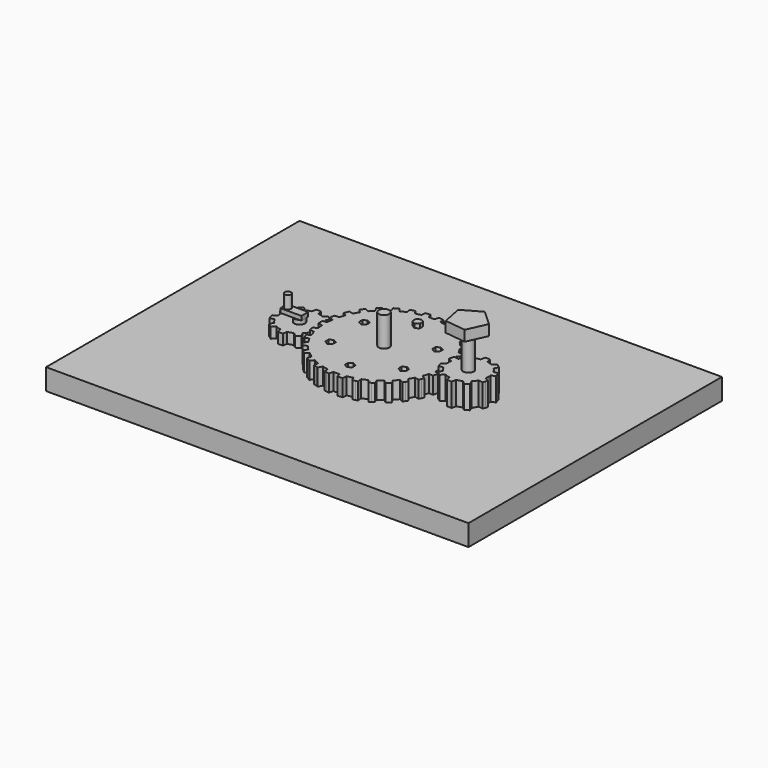
from build123d import *

# Parameters (mm, degrees)
F0_W      = 200
F0_H      = 150
F1_DEPTH  = 10
F2_R      = 4
F2_R_2    = 2.5
F3_DEPTH  = 3
F4_DEPTH  = 10
F6_DEPTH  = 5
F7_DEPTH  = 25
F8_DEPTH  = 30
F10_DEPTH = 11
F11_W     = 10
F11_H     = 4
F12_DEPTH = 2
F13_R     = 1.5
F14_DEPTH = 6
F16_DEPTH = 5
F18_DEPTH = 8
F20_DEPTH = 3
F21_DEPTH = 5


with BuildPart() as f1:
    # F0 (on Top) → F1 (new body)
    with BuildSketch(Plane.XY):
        Rectangle(F0_W, F0_H)
    extrude(amount=F1_DEPTH)

    # F2 (on face) → F3 (join)
    with BuildSketch(Plane.XY.offset(10)):
        Circle(F2_R)
        Circle(F2_R_2, mode=Mode.SUBTRACT)
        with Locations((-40, 0)):
            Circle(F2_R)
        with Locations((-40, 0)):
            Circle(F2_R_2, mode=Mode.SUBTRACT)
        with Locations((40, 0)):
            Circle(F2_R)
        with Locations((40, 0)):
            Circle(F2_R_2, mode=Mode.SUBTRACT)
    extrude(amount=F3_DEPTH)


with BuildPart() as f4:
    # F4 (new): a face of the model
    f4_faces = [f1.part.faces().sort_by_distance(p)[0] for p in [
        (-40, 0, 10),
    ]]
    extrude(f4_faces, amount=F4_DEPTH)

    # F5 (on face) → F6 (join)
    with BuildSketch(Plane.XY.offset(13)):
        with BuildLine():
            ThreePointArc((-30.7270362333, -1.3794085621), (-30.6505438577, -0.6915886375), (-30.625, 0))
            ThreePointArc((-30.625, 0), (-30.6505438577, 0.6915886375), (-30.7270362333, 1.3794085621))
            ThreePointArc((-30.7270362333, 1.3794085621), (-31.0838451597, 2.8970343223), (-31.6872187148, 4.3345463782))
            ThreePointArc((-31.6872187148, 4.3345463782), (-32.4154656777, 5.5104867402), (-33.3088107342, 6.566476316))
            ThreePointArc((-33.3088107342, 6.566476316), (-34.4895132598, 7.5845343223), (-35.8226011062, 8.3928519278))
            ThreePointArc((-35.8226011062, 8.3928519278), (-37.1029656777, 8.9161548403), (-38.4463921095, 9.2453733036))
            ThreePointArc((-38.4463921095, 9.2453733036), (-40, 9.375), (-41.5536078905, 9.2453733036))
            ThreePointArc((-41.5536078905, 9.2453733036), (-42.8970343223, 8.9161548403), (-44.1773988938, 8.3928519278))
            ThreePointArc((-44.1773988938, 8.3928519278), (-45.5104867402, 7.5845343223), (-46.6911892658, 6.566476316))
            ThreePointArc((-46.6911892658, 6.566476316), (-47.5845343223, 5.5104867402), (-48.3127812852, 4.3345463782))
            ThreePointArc((-48.3127812852, 4.3345463782), (-48.9161548403, 2.8970343223), (-49.2729637667, 1.3794085621))
            ThreePointArc((-49.2729637667, 1.3794085621), (-49.375, 0), (-49.2729637667, -1.3794085621))
            ThreePointArc((-49.2729637667, -1.3794085621), (-48.9161548403, -2.8970343223), (-48.3127812852, -4.3345463782))
            ThreePointArc((-48.3127812852, -4.3345463782), (-47.5845343223, -5.5104867402), (-46.6911892658, -6.566476316))
            ThreePointArc((-46.6911892658, -6.566476316), (-45.5104867402, -7.5845343223), (-44.1773988938, -8.3928519278))
            ThreePointArc((-44.1773988938, -8.3928519278), (-42.8970343223, -8.9161548403), (-41.5536078905, -9.2453733036))
            ThreePointArc((-41.5536078905, -9.2453733036), (-40, -9.375), (-38.4463921095, -9.2453733036))
            ThreePointArc((-38.4463921095, -9.2453733036), (-37.1029656777, -8.9161548403), (-35.8226011062, -8.3928519278))
            ThreePointArc((-35.8226011062, -8.3928519278), (-34.4895132598, -7.5845343223), (-33.3088107342, -6.566476316))
            ThreePointArc((-33.3088107342, -6.566476316), (-32.4154656777, -5.5104867402), (-31.6872187148, -4.3345463782))
            ThreePointArc((-31.6872187148, -4.3345463782), (-31.0838451597, -2.8970343223), (-30.7270362333, -1.3794085621))
        make_face()
        with BuildLine():
            ThreePointArc((-31.6872187148, 4.3345463782), (-31.0838451597, 2.8970343223), (-30.7270362333, 1.3794085621))
            Line((-30.7270362333, 1.3794085621), (-28.8176800574, 2.3946312492))
            Line((-28.8176800574, 2.3946312492), (-29.1817321271, 3.515068311))
            Line((-29.1817321271, 3.515068311), (-29.5457841969, 4.6355053728))
            Line((-29.5457841969, 4.6355053728), (-31.6872187148, 4.3345463782))
        make_face()
        with BuildLine():
            Line((-28.8176800574, -2.3946312492), (-30.7270362333, -1.3794085621))
            ThreePointArc((-30.7270362333, -1.3794085621), (-31.0838451597, -2.8970343223), (-31.6872187148, -4.3345463782))
            Line((-31.6872187148, -4.3345463782), (-29.5457841969, -4.6355053728))
            Line((-29.5457841969, -4.6355053728), (-29.1817321271, -3.515068311))
            Line((-29.1817321271, -3.515068311), (-28.8176800574, -2.3946312492))
        make_face()
        with BuildLine():
            ThreePointArc((-35.8226011062, 8.3928519278), (-34.4895132598, 7.5845343223), (-33.3088107342, 6.566476316))
            Line((-33.3088107342, 6.566476316), (-32.3608420629, 8.5101001246))
            Line((-32.3608420629, 8.5101001246), (-33.3139427552, 9.202568311))
            Line((-33.3139427552, 9.202568311), (-34.2670434475, 9.8950364974))
            Line((-34.2670434475, 9.8950364974), (-35.8226011062, 8.3928519278))
        make_face()
        with BuildLine():
            Line((-32.3608420629, -8.5101001246), (-33.3088107342, -6.566476316))
            ThreePointArc((-33.3088107342, -6.566476316), (-34.4895132598, -7.5845343223), (-35.8226011062, -8.3928519278))
            Line((-35.8226011062, -8.3928519278), (-34.2670434475, -9.8950364974))
            Line((-34.2670434475, -9.8950364974), (-33.3139427552, -9.202568311))
            Line((-33.3139427552, -9.202568311), (-32.3608420629, -8.5101001246))
        make_face()
        with BuildLine():
            ThreePointArc((-41.5536078905, 9.2453733036), (-40, 9.375), (-38.4463921095, 9.2453733036))
            Line((-38.4463921095, 9.2453733036), (-38.8219027549, 11.375))
            Line((-38.8219027549, 11.375), (-40, 11.375))
            Line((-40, 11.375), (-41.1780972451, 11.375))
            Line((-41.1780972451, 11.375), (-41.5536078905, 9.2453733036))
        make_face()
        with BuildLine():
            Line((-38.8219027549, -11.375), (-38.4463921095, -9.2453733036))
            ThreePointArc((-38.4463921095, -9.2453733036), (-40, -9.375), (-41.5536078905, -9.2453733036))
            Line((-41.5536078905, -9.2453733036), (-41.1780972451, -11.375))
            Line((-41.1780972451, -11.375), (-40, -11.375))
            Line((-40, -11.375), (-38.8219027549, -11.375))
        make_face()
        with BuildLine():
            ThreePointArc((-46.6911892658, 6.566476316), (-45.5104867402, 7.5845343223), (-44.1773988938, 8.3928519278))
            Line((-44.1773988938, 8.3928519278), (-45.7329565525, 9.8950364974))
            Line((-45.7329565525, 9.8950364974), (-46.6860572448, 9.202568311))
            Line((-46.6860572448, 9.202568311), (-47.6391579371, 8.5101001246))
            Line((-47.6391579371, 8.5101001246), (-46.6911892658, 6.566476316))
        make_face()
        with BuildLine():
            Line((-45.7329565525, -9.8950364974), (-44.1773988938, -8.3928519278))
            ThreePointArc((-44.1773988938, -8.3928519278), (-45.5104867402, -7.5845343223), (-46.6911892658, -6.566476316))
            Line((-46.6911892658, -6.566476316), (-47.6391579371, -8.5101001246))
            Line((-47.6391579371, -8.5101001246), (-46.6860572448, -9.202568311))
            Line((-46.6860572448, -9.202568311), (-45.7329565525, -9.8950364974))
        make_face()
        with BuildLine():
            ThreePointArc((-49.2729637667, 1.3794085621), (-48.9161548403, 2.8970343223), (-48.3127812852, 4.3345463782))
            Line((-48.3127812852, 4.3345463782), (-50.4542158031, 4.6355053728))
            Line((-50.4542158031, 4.6355053728), (-50.8182678729, 3.515068311))
            Line((-50.8182678729, 3.515068311), (-51.1823199426, 2.3946312492))
            Line((-51.1823199426, 2.3946312492), (-49.2729637667, 1.3794085621))
        make_face()
        with BuildLine():
            Line((-50.4542158031, -4.6355053728), (-48.3127812852, -4.3345463782))
            ThreePointArc((-48.3127812852, -4.3345463782), (-48.9161548403, -2.8970343223), (-49.2729637667, -1.3794085621))
            Line((-49.2729637667, -1.3794085621), (-51.1823199426, -2.3946312492))
            Line((-51.1823199426, -2.3946312492), (-50.8182678729, -3.515068311))
            Line((-50.8182678729, -3.515068311), (-50.4542158031, -4.6355053728))
        make_face()
    extrude(amount=F6_DEPTH)

    # F11 (on face) → F12 (join)
    with BuildSketch(Plane.XY.offset(20)):
        with Locations((-42.5, 0)):
            Rectangle(F11_W, F11_H)
    extrude(amount=F12_DEPTH)

    # F13 (on face) → F14 (join)
    with BuildSketch(Plane.XY.offset(22)):
        with Locations((-45.5, 0)):
            Circle(F13_R)
    extrude(amount=F14_DEPTH)


with BuildPart() as f7:
    # F7 (new): a face of the model
    f7_faces = [f1.part.faces().sort_by_distance(p)[0] for p in [
        (0, 0, 10),
    ]]
    extrude(f7_faces, amount=F7_DEPTH)

    # F17 (on face) → F18 (join)
    with BuildSketch(Plane.XY.offset(13)):
        with BuildLine():
            ThreePointArc((28.0829066802, -1.5381733945), (28.1144747006, -0.7693746225), (28.125, 0))
            ThreePointArc((28.125, 0), (28.1144747006, 0.7693746225), (28.0829066802, 1.5381733945))
            ThreePointArc((28.0829066802, 1.5381733945), (27.9709283072, 2.9398630294), (27.7890320221, 4.3342039956))
            ThreePointArc((27.7890320221, 4.3342039956), (27.5104012706, 5.8475163042), (27.1494235596, 7.3433252263))
            ThreePointArc((27.1494235596, 7.3433252263), (26.7484645208, 8.6911029668), (26.280643318, 10.0171558733))
            ThreePointArc((26.280643318, 10.0171558733), (25.6934659962, 11.4394680865), (25.0293803521, 12.8275385085))
            ThreePointArc((25.0293803521, 12.8275385085), (24.3569644814, 14.0625), (23.6236643925, 15.2623099717))
            ThreePointArc((23.6236643925, 15.2623099717), (22.7536029668, 16.5314602207), (21.815433119, 17.7511268046))
            ThreePointArc((21.815433119, 17.7511268046), (20.9009482166, 18.8192983038), (19.934217974, 19.8404278876))
            ThreePointArc((19.934217974, 19.8404278876), (18.8192983038, 20.9009482166), (17.6480467764, 21.8989056799))
            ThreePointArc((17.6480467764, 21.8989056799), (16.5314602207, 22.7536029668), (15.3735505752, 23.5514238999))
            ThreePointArc((15.3735505752, 23.5514238999), (14.0625, 24.3569644814), (12.709356105, 25.0895972944))
            ThreePointArc((12.709356105, 25.0895972944), (11.4394680865, 25.6934659962), (10.1409852457, 26.2331096755))
            ThreePointArc((10.1409852457, 26.2331096755), (8.6911029668, 26.7484645208), (7.2152055856, 27.1837531139))
            ThreePointArc((7.2152055856, 27.1837531139), (5.8475163042, 27.5104012706), (4.4652101991, 27.7682826779))
            ThreePointArc((4.4652101991, 27.7682826779), (2.9398630294, 27.9709283072), (1.4057159597, 28.0898484802))
            ThreePointArc((1.4057159597, 28.0898484802), (0, 28.125), (-1.4057159597, 28.0898484802))
            ThreePointArc((-1.4057159597, 28.0898484802), (-2.9398630294, 27.9709283072), (-4.4652101991, 27.7682826779))
            ThreePointArc((-4.4652101991, 27.7682826779), (-5.8475163042, 27.5104012706), (-7.2152055856, 27.1837531139))
            ThreePointArc((-7.2152055856, 27.1837531139), (-8.6911029668, 26.7484645208), (-10.1409852457, 26.2331096755))
            ThreePointArc((-10.1409852457, 26.2331096755), (-11.4394680865, 25.6934659962), (-12.709356105, 25.0895972944))
            ThreePointArc((-12.709356105, 25.0895972944), (-14.0625, 24.3569644814), (-15.3735505752, 23.5514238999))
            ThreePointArc((-15.3735505752, 23.5514238999), (-16.5314602207, 22.7536029668), (-17.6480467764, 21.8989056799))
            ThreePointArc((-17.6480467764, 21.8989056799), (-18.8192983038, 20.9009482166), (-19.934217974, 19.8404278876))
            ThreePointArc((-19.934217974, 19.8404278876), (-20.9009482166, 18.8192983038), (-21.815433119, 17.7511268046))
            ThreePointArc((-21.815433119, 17.7511268046), (-22.7536029668, 16.5314602207), (-23.6236643925, 15.2623099717))
            ThreePointArc((-23.6236643925, 15.2623099717), (-24.3569644814, 14.0625), (-25.0293803521, 12.8275385085))
            ThreePointArc((-25.0293803521, 12.8275385085), (-25.6934659962, 11.4394680865), (-26.280643318, 10.0171558733))
            ThreePointArc((-26.280643318, 10.0171558733), (-26.7484645208, 8.6911029668), (-27.1494235596, 7.3433252263))
            ThreePointArc((-27.1494235596, 7.3433252263), (-27.5104012706, 5.8475163042), (-27.7890320221, 4.3342039956))
            ThreePointArc((-27.7890320221, 4.3342039956), (-27.9709283072, 2.9398630294), (-28.0829066802, 1.5381733945))
            ThreePointArc((-28.0829066802, 1.5381733945), (-28.125, 0), (-28.0829066802, -1.5381733945))
            ThreePointArc((-28.0829066802, -1.5381733945), (-27.9709283072, -2.9398630294), (-27.7890320221, -4.3342039956))
            ThreePointArc((-27.7890320221, -4.3342039956), (-27.5104012706, -5.8475163042), (-27.1494235596, -7.3433252263))
            ThreePointArc((-27.1494235596, -7.3433252263), (-26.7484645208, -8.6911029668), (-26.280643318, -10.0171558733))
            ThreePointArc((-26.280643318, -10.0171558733), (-25.6934659962, -11.4394680865), (-25.0293803521, -12.8275385085))
            ThreePointArc((-25.0293803521, -12.8275385085), (-24.3569644814, -14.0625), (-23.6236643925, -15.2623099717))
            ThreePointArc((-23.6236643925, -15.2623099717), (-22.7536029668, -16.5314602207), (-21.815433119, -17.7511268046))
            ThreePointArc((-21.815433119, -17.7511268046), (-20.9009482166, -18.8192983038), (-19.934217974, -19.8404278876))
            ThreePointArc((-19.934217974, -19.8404278876), (-18.8192983038, -20.9009482166), (-17.6480467764, -21.8989056799))
            ThreePointArc((-17.6480467764, -21.8989056799), (-16.5314602207, -22.7536029668), (-15.3735505752, -23.5514238999))
            ThreePointArc((-15.3735505752, -23.5514238999), (-14.0625, -24.3569644814), (-12.709356105, -25.0895972944))
            ThreePointArc((-12.709356105, -25.0895972944), (-11.4394680865, -25.6934659962), (-10.1409852457, -26.2331096755))
            ThreePointArc((-10.1409852457, -26.2331096755), (-8.6911029668, -26.7484645208), (-7.2152055856, -27.1837531139))
            ThreePointArc((-7.2152055856, -27.1837531139), (-5.8475163042, -27.5104012706), (-4.4652101991, -27.7682826779))
            ThreePointArc((-4.4652101991, -27.7682826779), (-2.9398630294, -27.9709283072), (-1.4057159597, -28.0898484802))
            ThreePointArc((-1.4057159597, -28.0898484802), (0, -28.125), (1.4057159597, -28.0898484802))
            ThreePointArc((1.4057159597, -28.0898484802), (2.9398630294, -27.9709283072), (4.4652101991, -27.7682826779))
            ThreePointArc((4.4652101991, -27.7682826779), (5.8475163042, -27.5104012706), (7.2152055856, -27.1837531139))
            ThreePointArc((7.2152055856, -27.1837531139), (8.6911029668, -26.7484645208), (10.1409852457, -26.2331096755))
            ThreePointArc((10.1409852457, -26.2331096755), (11.4394680865, -25.6934659962), (12.709356105, -25.0895972944))
            ThreePointArc((12.709356105, -25.0895972944), (14.0625, -24.3569644814), (15.3735505752, -23.5514238999))
            ThreePointArc((15.3735505752, -23.5514238999), (16.5314602207, -22.7536029668), (17.6480467764, -21.8989056799))
            ThreePointArc((17.6480467764, -21.8989056799), (18.8192983038, -20.9009482166), (19.934217974, -19.8404278876))
            ThreePointArc((19.934217974, -19.8404278876), (20.9009482166, -18.8192983038), (21.815433119, -17.7511268046))
            ThreePointArc((21.815433119, -17.7511268046), (22.7536029668, -16.5314602207), (23.6236643925, -15.2623099717))
            ThreePointArc((23.6236643925, -15.2623099717), (24.3569644814, -14.0625), (25.0293803521, -12.8275385085))
            ThreePointArc((25.0293803521, -12.8275385085), (25.6934659962, -11.4394680865), (26.280643318, -10.0171558733))
            ThreePointArc((26.280643318, -10.0171558733), (26.7484645208, -8.6911029668), (27.1494235596, -7.3433252263))
            ThreePointArc((27.1494235596, -7.3433252263), (27.5104012706, -5.8475163042), (27.7890320221, -4.3342039956))
            ThreePointArc((27.7890320221, -4.3342039956), (27.9709283072, -2.9398630294), (28.0829066802, -1.5381733945))
        make_face()
        with BuildLine():
            ThreePointArc((28.0829066802, 1.5381733945), (28.1144747006, 0.7693746225), (28.125, 0))
            ThreePointArc((28.125, 0), (28.1144747006, -0.7693746225), (28.0829066802, -1.5381733945))
            Line((28.0829066802, -1.5381733945), (30.125, -1.1780972451))
            Line((30.125, -1.1780972451), (30.125, 0))
            Line((30.125, 0), (30.125, 1.1780972451))
            Line((30.125, 1.1780972451), (28.0829066802, 1.5381733945))
        make_face()
        with BuildLine():
            ThreePointArc((27.1494235596, 7.3433252263), (27.5104012706, 5.8475163042), (27.7890320221, 4.3342039956))
            Line((27.7890320221, 4.3342039956), (29.7116366623, 5.1109866922))
            Line((29.7116366623, 5.1109866922), (29.4666964721, 6.2633396859))
            Line((29.4666964721, 6.2633396859), (29.2217562819, 7.4156926796))
            Line((29.2217562819, 7.4156926796), (27.1494235596, 7.3433252263))
        make_face()
        with BuildLine():
            Line((29.7116366623, -5.1109866922), (27.7890320221, -4.3342039956))
            ThreePointArc((27.7890320221, -4.3342039956), (27.5104012706, -5.8475163042), (27.1494235596, -7.3433252263))
            Line((27.1494235596, -7.3433252263), (29.2217562819, -7.4156926796))
            Line((29.2217562819, -7.4156926796), (29.4666964721, -6.2633396859))
            Line((29.4666964721, -6.2633396859), (29.7116366623, -5.1109866922))
        make_face()
        with BuildLine():
            ThreePointArc((25.0293803521, 12.8275385085), (25.6934659962, 11.4394680865), (26.280643318, 10.0171558733))
            Line((26.280643318, 10.0171558733), (27.9997322302, 11.1766959857))
            Line((27.9997322302, 11.1766959857), (27.5205569115, 12.2529413727))
            Line((27.5205569115, 12.2529413727), (27.0413815928, 13.3291867596))
            Line((27.0413815928, 13.3291867596), (25.0293803521, 12.8275385085))
        make_face()
        with BuildLine():
            Line((27.9997322302, -11.1766959857), (26.280643318, -10.0171558733))
            ThreePointArc((26.280643318, -10.0171558733), (25.6934659962, -11.4394680865), (25.0293803521, -12.8275385085))
            Line((25.0293803521, -12.8275385085), (27.0413815928, -13.3291867596))
            Line((27.0413815928, -13.3291867596), (27.5205569115, -12.2529413727))
            Line((27.5205569115, -12.2529413727), (27.9997322302, -11.1766959857))
        make_face()
        with BuildLine():
            ThreePointArc((21.815433119, 17.7511268046), (22.7536029668, 16.5314602207), (23.6236643925, 15.2623099717))
            Line((23.6236643925, 15.2623099717), (25.064105142, 16.753930033))
            Line((25.064105142, 16.753930033), (24.3716369555, 17.7070307253))
            Line((24.3716369555, 17.7070307253), (23.6791687691, 18.6601314176))
            Line((23.6791687691, 18.6601314176), (21.815433119, 17.7511268046))
        make_face()
        with BuildLine():
            Line((25.064105142, -16.753930033), (23.6236643925, -15.2623099717))
            ThreePointArc((23.6236643925, -15.2623099717), (22.7536029668, -16.5314602207), (21.815433119, -17.7511268046))
            Line((21.815433119, -17.7511268046), (23.6791687691, -18.6601314176))
            Line((23.6791687691, -18.6601314176), (24.3716369555, -17.7070307253))
            Line((24.3716369555, -17.7070307253), (25.064105142, -16.753930033))
        make_face()
        with BuildLine():
            ThreePointArc((17.6480467764, 21.8989056799), (18.8192983038, 20.9009482166), (19.934217974, 19.8404278876))
            Line((19.934217974, 19.8404278876), (21.0330563882, 21.5989369435))
            Line((21.0330563882, 21.5989369435), (20.1575595166, 22.3872378675))
            Line((20.1575595166, 22.3872378675), (19.282062645, 23.1755387915))
            Line((19.282062645, 23.1755387915), (17.6480467764, 21.8989056799))
        make_face()
        with BuildLine():
            Line((21.0330563882, -21.5989369435), (19.934217974, -19.8404278876))
            ThreePointArc((19.934217974, -19.8404278876), (18.8192983038, -20.9009482166), (17.6480467764, -21.8989056799))
            Line((17.6480467764, -21.8989056799), (19.282062645, -23.1755387915))
            Line((19.282062645, -23.1755387915), (20.1575595166, -22.3872378675))
            Line((20.1575595166, -22.3872378675), (21.0330563882, -21.5989369435))
        make_face()
        with BuildLine():
            ThreePointArc((12.709356105, 25.0895972944), (14.0625, 24.3569644814), (15.3735505752, 23.5514238999))
            Line((15.3735505752, 23.5514238999), (16.0827621424, 25.4999666665))
            Line((16.0827621424, 25.4999666665), (15.0625, 26.089015289))
            Line((15.0625, 26.089015289), (14.0422378576, 26.6780639116))
            Line((14.0422378576, 26.6780639116), (12.709356105, 25.0895972944))
        make_face()
        with BuildLine():
            Line((16.0827621424, -25.4999666665), (15.3735505752, -23.5514238999))
            ThreePointArc((15.3735505752, -23.5514238999), (14.0625, -24.3569644814), (12.709356105, -25.0895972944))
            Line((12.709356105, -25.0895972944), (14.0422378576, -26.6780639116))
            Line((14.0422378576, -26.6780639116), (15.0625, -26.089015289))
            Line((15.0625, -26.089015289), (16.0827621424, -25.4999666665))
        make_face()
        with BuildLine():
            ThreePointArc((7.2152055856, 27.1837531139), (8.6911029668, 26.7484645208), (10.1409852457, 26.2331096755))
            Line((10.1409852457, 26.2331096755), (10.4295740173, 28.2865254836))
            Line((10.4295740173, 28.2865254836), (9.3091369555, 28.6505775534))
            Line((9.3091369555, 28.6505775534), (8.1886998938, 29.0146296232))
            Line((8.1886998938, 29.0146296232), (7.2152055856, 27.1837531139))
        make_face()
        with BuildLine():
            Line((10.4295740173, -28.2865254836), (10.1409852457, -26.2331096755))
            ThreePointArc((10.1409852457, -26.2331096755), (8.6911029668, -26.7484645208), (7.2152055856, -27.1837531139))
            Line((7.2152055856, -27.1837531139), (8.1886998938, -29.0146296232))
            Line((8.1886998938, -29.0146296232), (9.3091369555, -28.6505775534))
            Line((9.3091369555, -28.6505775534), (10.4295740173, -28.2865254836))
        make_face()
        with BuildLine():
            ThreePointArc((1.4057159597, 28.0898484802), (2.9398630294, 27.9709283072), (4.4652101991, 27.7682826779))
            Line((4.4652101991, 27.7682826779), (4.3205634611, 29.8368274034))
            Line((4.3205634611, 29.8368274034), (3.1489199559, 29.959972098))
            Line((3.1489199559, 29.959972098), (1.9772764508, 30.0831167926))
            Line((1.9772764508, 30.0831167926), (1.4057159597, 28.0898484802))
        make_face()
        with BuildLine():
            Line((4.3205634611, -29.8368274034), (4.4652101991, -27.7682826779))
            ThreePointArc((4.4652101991, -27.7682826779), (2.9398630294, -27.9709283072), (1.4057159597, -28.0898484802))
            Line((1.4057159597, -28.0898484802), (1.9772764508, -30.0831167926))
            Line((1.9772764508, -30.0831167926), (3.1489199559, -29.959972098))
            Line((3.1489199559, -29.959972098), (4.3205634611, -29.8368274034))
        make_face()
        with BuildLine():
            ThreePointArc((-4.4652101991, 27.7682826779), (-2.9398630294, 27.9709283072), (-1.4057159597, 28.0898484802))
            Line((-1.4057159597, 28.0898484802), (-1.9772764508, 30.0831167926))
            Line((-1.9772764508, 30.0831167926), (-3.1489199559, 29.959972098))
            Line((-3.1489199559, 29.959972098), (-4.3205634611, 29.8368274034))
            Line((-4.3205634611, 29.8368274034), (-4.4652101991, 27.7682826779))
        make_face()
        with BuildLine():
            Line((-1.9772764508, -30.0831167926), (-1.4057159597, -28.0898484802))
            ThreePointArc((-1.4057159597, -28.0898484802), (-2.9398630294, -27.9709283072), (-4.4652101991, -27.7682826779))
            Line((-4.4652101991, -27.7682826779), (-4.3205634611, -29.8368274034))
            Line((-4.3205634611, -29.8368274034), (-3.1489199559, -29.959972098))
            Line((-3.1489199559, -29.959972098), (-1.9772764508, -30.0831167926))
        make_face()
        with BuildLine():
            ThreePointArc((-10.1409852457, 26.2331096755), (-8.6911029668, 26.7484645208), (-7.2152055856, 27.1837531139))
            Line((-7.2152055856, 27.1837531139), (-8.1886998938, 29.0146296232))
            Line((-8.1886998938, 29.0146296232), (-9.3091369555, 28.6505775534))
            Line((-9.3091369555, 28.6505775534), (-10.4295740173, 28.2865254836))
            Line((-10.4295740173, 28.2865254836), (-10.1409852457, 26.2331096755))
        make_face()
        with BuildLine():
            Line((-8.1886998938, -29.0146296232), (-7.2152055856, -27.1837531139))
            ThreePointArc((-7.2152055856, -27.1837531139), (-8.6911029668, -26.7484645208), (-10.1409852457, -26.2331096755))
            Line((-10.1409852457, -26.2331096755), (-10.4295740173, -28.2865254836))
            Line((-10.4295740173, -28.2865254836), (-9.3091369555, -28.6505775534))
            Line((-9.3091369555, -28.6505775534), (-8.1886998938, -29.0146296232))
        make_face()
        with BuildLine():
            ThreePointArc((-15.3735505752, 23.5514238999), (-14.0625, 24.3569644814), (-12.709356105, 25.0895972944))
            Line((-12.709356105, 25.0895972944), (-14.0422378576, 26.6780639116))
            Line((-14.0422378576, 26.6780639116), (-15.0625, 26.089015289))
            Line((-15.0625, 26.089015289), (-16.0827621424, 25.4999666665))
            Line((-16.0827621424, 25.4999666665), (-15.3735505752, 23.5514238999))
        make_face()
        with BuildLine():
            Line((-14.0422378576, -26.6780639116), (-12.709356105, -25.0895972944))
            ThreePointArc((-12.709356105, -25.0895972944), (-14.0625, -24.3569644814), (-15.3735505752, -23.5514238999))
            Line((-15.3735505752, -23.5514238999), (-16.0827621424, -25.4999666665))
            Line((-16.0827621424, -25.4999666665), (-15.0625, -26.089015289))
            Line((-15.0625, -26.089015289), (-14.0422378576, -26.6780639116))
        make_face()
        with BuildLine():
            ThreePointArc((-19.934217974, 19.8404278876), (-18.8192983038, 20.9009482166), (-17.6480467764, 21.8989056799))
            Line((-17.6480467764, 21.8989056799), (-19.282062645, 23.1755387915))
            Line((-19.282062645, 23.1755387915), (-20.1575595166, 22.3872378675))
            Line((-20.1575595166, 22.3872378675), (-21.0330563882, 21.5989369435))
            Line((-21.0330563882, 21.5989369435), (-19.934217974, 19.8404278876))
        make_face()
        with BuildLine():
            Line((-19.282062645, -23.1755387915), (-17.6480467764, -21.8989056799))
            ThreePointArc((-17.6480467764, -21.8989056799), (-18.8192983038, -20.9009482166), (-19.934217974, -19.8404278876))
            Line((-19.934217974, -19.8404278876), (-21.0330563882, -21.5989369435))
            Line((-21.0330563882, -21.5989369435), (-20.1575595166, -22.3872378675))
            Line((-20.1575595166, -22.3872378675), (-19.282062645, -23.1755387915))
        make_face()
        with BuildLine():
            ThreePointArc((-23.6236643925, 15.2623099717), (-22.7536029668, 16.5314602207), (-21.815433119, 17.7511268046))
            Line((-21.815433119, 17.7511268046), (-23.6791687691, 18.6601314176))
            Line((-23.6791687691, 18.6601314176), (-24.3716369555, 17.7070307253))
            Line((-24.3716369555, 17.7070307253), (-25.064105142, 16.753930033))
            Line((-25.064105142, 16.753930033), (-23.6236643925, 15.2623099717))
        make_face()
        with BuildLine():
            Line((-23.6791687691, -18.6601314176), (-21.815433119, -17.7511268046))
            ThreePointArc((-21.815433119, -17.7511268046), (-22.7536029668, -16.5314602207), (-23.6236643925, -15.2623099717))
            Line((-23.6236643925, -15.2623099717), (-25.064105142, -16.753930033))
            Line((-25.064105142, -16.753930033), (-24.3716369555, -17.7070307253))
            Line((-24.3716369555, -17.7070307253), (-23.6791687691, -18.6601314176))
        make_face()
        with BuildLine():
            ThreePointArc((-26.280643318, 10.0171558733), (-25.6934659962, 11.4394680865), (-25.0293803521, 12.8275385085))
            Line((-25.0293803521, 12.8275385085), (-27.0413815928, 13.3291867596))
            Line((-27.0413815928, 13.3291867596), (-27.5205569115, 12.2529413727))
            Line((-27.5205569115, 12.2529413727), (-27.9997322302, 11.1766959857))
            Line((-27.9997322302, 11.1766959857), (-26.280643318, 10.0171558733))
        make_face()
        with BuildLine():
            Line((-27.0413815928, -13.3291867596), (-25.0293803521, -12.8275385085))
            ThreePointArc((-25.0293803521, -12.8275385085), (-25.6934659962, -11.4394680865), (-26.280643318, -10.0171558733))
            Line((-26.280643318, -10.0171558733), (-27.9997322302, -11.1766959857))
            Line((-27.9997322302, -11.1766959857), (-27.5205569115, -12.2529413727))
            Line((-27.5205569115, -12.2529413727), (-27.0413815928, -13.3291867596))
        make_face()
        with BuildLine():
            ThreePointArc((-27.7890320221, 4.3342039956), (-27.5104012706, 5.8475163042), (-27.1494235596, 7.3433252263))
            Line((-27.1494235596, 7.3433252263), (-29.2217562819, 7.4156926796))
            Line((-29.2217562819, 7.4156926796), (-29.4666964721, 6.2633396859))
            Line((-29.4666964721, 6.2633396859), (-29.7116366623, 5.1109866922))
            Line((-29.7116366623, 5.1109866922), (-27.7890320221, 4.3342039956))
        make_face()
        with BuildLine():
            Line((-29.2217562819, -7.4156926796), (-27.1494235596, -7.3433252263))
            ThreePointArc((-27.1494235596, -7.3433252263), (-27.5104012706, -5.8475163042), (-27.7890320221, -4.3342039956))
            Line((-27.7890320221, -4.3342039956), (-29.7116366623, -5.1109866922))
            Line((-29.7116366623, -5.1109866922), (-29.4666964721, -6.2633396859))
            Line((-29.4666964721, -6.2633396859), (-29.2217562819, -7.4156926796))
        make_face()
        with BuildLine():
            ThreePointArc((-28.0829066802, -1.5381733945), (-28.125, 0), (-28.0829066802, 1.5381733945))
            Line((-28.0829066802, 1.5381733945), (-30.125, 1.1780972451))
            Line((-30.125, 1.1780972451), (-30.125, 0))
            Line((-30.125, 0), (-30.125, -1.1780972451))
            Line((-30.125, -1.1780972451), (-28.0829066802, -1.5381733945))
        make_face()
    extrude(amount=F18_DEPTH)

    # F19 (on face) → F20 (cut)
    with BuildSketch(Plane.XY.offset(21)):
        Polygon((0, 22), (-1.7320508076, 21), (-1.7320508076, 19), (0, 18), (1.7320508076, 19), (1.7320508076, 21), align=None)
        Polygon((-19.0525588833, 11), (-19.0525588833, 9), (-17.3205080757, 8), (-15.5884572681, 9), (-15.5884572681, 11), (-17.3205080757, 12), align=None)
        Polygon((-19.0525588833, -11), (-17.3205080757, -12), (-15.5884572681, -11), (-15.5884572681, -9), (-17.3205080757, -8), (-19.0525588833, -9), align=None)
        Polygon((0, -22), (1.7320508076, -21), (1.7320508076, -19), (0, -18), (-1.7320508076, -19), (-1.7320508076, -21), align=None)
        Polygon((19.0525588833, -11), (19.0525588833, -9), (17.3205080757, -8), (15.5884572681, -9), (15.5884572681, -11), (17.3205080757, -12), align=None)
        Polygon((19.0525588833, 11), (17.3205080757, 12), (15.5884572681, 11), (15.5884572681, 9), (17.3205080757, 8), (19.0525588833, 9), align=None)
    extrude(amount=-F20_DEPTH, mode=Mode.SUBTRACT)


with BuildPart() as f8:
    # F8 (new): a face of the model
    f8_faces = [f1.part.faces().sort_by_distance(p)[0] for p in [
        (40, 0, 10),
    ]]
    extrude(f8_faces, amount=F8_DEPTH)

    # F9 (on face) → F10 (join)
    with BuildSketch(Plane.XY.offset(13)):
        with BuildLine():
            ThreePointArc((49.2729637667, -1.3794085621), (49.3494561423, -0.6915886375), (49.375, 0))
            ThreePointArc((49.375, 0), (49.3494561423, 0.6915886375), (49.2729637667, 1.3794085621))
            ThreePointArc((49.2729637667, 1.3794085621), (48.9161548403, 2.8970343223), (48.3127812852, 4.3345463782))
            ThreePointArc((48.3127812852, 4.3345463782), (47.5845343223, 5.5104867402), (46.6911892658, 6.566476316))
            ThreePointArc((46.6911892658, 6.566476316), (45.5104867402, 7.5845343223), (44.1773988938, 8.3928519278))
            ThreePointArc((44.1773988938, 8.3928519278), (42.8970343223, 8.9161548403), (41.5536078905, 9.2453733036))
            ThreePointArc((41.5536078905, 9.2453733036), (40, 9.375), (38.4463921095, 9.2453733036))
            ThreePointArc((38.4463921095, 9.2453733036), (37.1029656777, 8.9161548403), (35.8226011062, 8.3928519278))
            ThreePointArc((35.8226011062, 8.3928519278), (34.4895132598, 7.5845343223), (33.3088107342, 6.566476316))
            ThreePointArc((33.3088107342, 6.566476316), (32.4154656777, 5.5104867402), (31.6872187148, 4.3345463782))
            ThreePointArc((31.6872187148, 4.3345463782), (31.0838451597, 2.8970343223), (30.7270362333, 1.3794085621))
            ThreePointArc((30.7270362333, 1.3794085621), (30.625, 0), (30.7270362333, -1.3794085621))
            ThreePointArc((30.7270362333, -1.3794085621), (31.0838451597, -2.8970343223), (31.6872187148, -4.3345463782))
            ThreePointArc((31.6872187148, -4.3345463782), (32.4154656777, -5.5104867402), (33.3088107342, -6.566476316))
            ThreePointArc((33.3088107342, -6.566476316), (34.4895132598, -7.5845343223), (35.8226011062, -8.3928519278))
            ThreePointArc((35.8226011062, -8.3928519278), (37.1029656777, -8.9161548403), (38.4463921095, -9.2453733036))
            ThreePointArc((38.4463921095, -9.2453733036), (40, -9.375), (41.5536078905, -9.2453733036))
            ThreePointArc((41.5536078905, -9.2453733036), (42.8970343223, -8.9161548403), (44.1773988938, -8.3928519278))
            ThreePointArc((44.1773988938, -8.3928519278), (45.5104867402, -7.5845343223), (46.6911892658, -6.566476316))
            ThreePointArc((46.6911892658, -6.566476316), (47.5845343223, -5.5104867402), (48.3127812852, -4.3345463782))
            ThreePointArc((48.3127812852, -4.3345463782), (48.9161548403, -2.8970343223), (49.2729637667, -1.3794085621))
        make_face()
        with BuildLine():
            ThreePointArc((48.3127812852, 4.3345463782), (48.9161548403, 2.8970343223), (49.2729637667, 1.3794085621))
            Line((49.2729637667, 1.3794085621), (51.1823199426, 2.3946312492))
            Line((51.1823199426, 2.3946312492), (50.8182678729, 3.515068311))
            Line((50.8182678729, 3.515068311), (50.4542158031, 4.6355053728))
            Line((50.4542158031, 4.6355053728), (48.3127812852, 4.3345463782))
        make_face()
        with BuildLine():
            Line((51.1823199426, -2.3946312492), (49.2729637667, -1.3794085621))
            ThreePointArc((49.2729637667, -1.3794085621), (48.9161548403, -2.8970343223), (48.3127812852, -4.3345463782))
            Line((48.3127812852, -4.3345463782), (50.4542158031, -4.6355053728))
            Line((50.4542158031, -4.6355053728), (50.8182678729, -3.515068311))
            Line((50.8182678729, -3.515068311), (51.1823199426, -2.3946312492))
        make_face()
        with BuildLine():
            ThreePointArc((44.1773988938, 8.3928519278), (45.5104867402, 7.5845343223), (46.6911892658, 6.566476316))
            Line((46.6911892658, 6.566476316), (47.6391579371, 8.5101001246))
            Line((47.6391579371, 8.5101001246), (46.6860572448, 9.202568311))
            Line((46.6860572448, 9.202568311), (45.7329565525, 9.8950364974))
            Line((45.7329565525, 9.8950364974), (44.1773988938, 8.3928519278))
        make_face()
        with BuildLine():
            Line((47.6391579371, -8.5101001246), (46.6911892658, -6.566476316))
            ThreePointArc((46.6911892658, -6.566476316), (45.5104867402, -7.5845343223), (44.1773988938, -8.3928519278))
            Line((44.1773988938, -8.3928519278), (45.7329565525, -9.8950364974))
            Line((45.7329565525, -9.8950364974), (46.6860572448, -9.202568311))
            Line((46.6860572448, -9.202568311), (47.6391579371, -8.5101001246))
        make_face()
        with BuildLine():
            ThreePointArc((38.4463921095, 9.2453733036), (40, 9.375), (41.5536078905, 9.2453733036))
            Line((41.5536078905, 9.2453733036), (41.1780972451, 11.375))
            Line((41.1780972451, 11.375), (40, 11.375))
            Line((40, 11.375), (38.8219027549, 11.375))
            Line((38.8219027549, 11.375), (38.4463921095, 9.2453733036))
        make_face()
        with BuildLine():
            Line((41.1780972451, -11.375), (41.5536078905, -9.2453733036))
            ThreePointArc((41.5536078905, -9.2453733036), (40, -9.375), (38.4463921095, -9.2453733036))
            Line((38.4463921095, -9.2453733036), (38.8219027549, -11.375))
            Line((38.8219027549, -11.375), (40, -11.375))
            Line((40, -11.375), (41.1780972451, -11.375))
        make_face()
        with BuildLine():
            ThreePointArc((33.3088107342, 6.566476316), (34.4895132598, 7.5845343223), (35.8226011062, 8.3928519278))
            Line((35.8226011062, 8.3928519278), (34.2670434475, 9.8950364974))
            Line((34.2670434475, 9.8950364974), (33.3139427552, 9.202568311))
            Line((33.3139427552, 9.202568311), (32.3608420629, 8.5101001246))
            Line((32.3608420629, 8.5101001246), (33.3088107342, 6.566476316))
        make_face()
        with BuildLine():
            Line((34.2670434475, -9.8950364974), (35.8226011062, -8.3928519278))
            ThreePointArc((35.8226011062, -8.3928519278), (34.4895132598, -7.5845343223), (33.3088107342, -6.566476316))
            Line((33.3088107342, -6.566476316), (32.3608420629, -8.5101001246))
            Line((32.3608420629, -8.5101001246), (33.3139427552, -9.202568311))
            Line((33.3139427552, -9.202568311), (34.2670434475, -9.8950364974))
        make_face()
        with BuildLine():
            ThreePointArc((30.7270362333, 1.3794085621), (31.0838451597, 2.8970343223), (31.6872187148, 4.3345463782))
            Line((31.6872187148, 4.3345463782), (29.5457841969, 4.6355053728))
            Line((29.5457841969, 4.6355053728), (29.1817321271, 3.515068311))
            Line((29.1817321271, 3.515068311), (28.8176800574, 2.3946312492))
            Line((28.8176800574, 2.3946312492), (30.7270362333, 1.3794085621))
        make_face()
        with BuildLine():
            Line((29.5457841969, -4.6355053728), (31.6872187148, -4.3345463782))
            ThreePointArc((31.6872187148, -4.3345463782), (31.0838451597, -2.8970343223), (30.7270362333, -1.3794085621))
            Line((30.7270362333, -1.3794085621), (28.8176800574, -2.3946312492))
            Line((28.8176800574, -2.3946312492), (29.1817321271, -3.515068311))
            Line((29.1817321271, -3.515068311), (29.5457841969, -4.6355053728))
        make_face()
    extrude(amount=F10_DEPTH)

    # F15 (on face) → F16 (join)
    with BuildSketch(Plane.XY.offset(40)):
        Polygon((40.9886944172, 8.4488557287), (32.2701840811, 3.5511442713), (34.2340166182, -6.2541278701), (44.1662422103, -7.416407865), (48.3408626732, 1.6705357351), align=None)
    extrude(amount=F16_DEPTH)


with BuildPart() as f21:
    # F21 (new): a face of the model
    f21_faces = [f7.part.faces().sort_by_distance(p)[0] for p in [
        (0, 20, 18),
    ]]
    extrude(f21_faces, amount=F21_DEPTH)


solid = Compound([f1.part, f4.part, f7.part, f8.part, f21.part])
